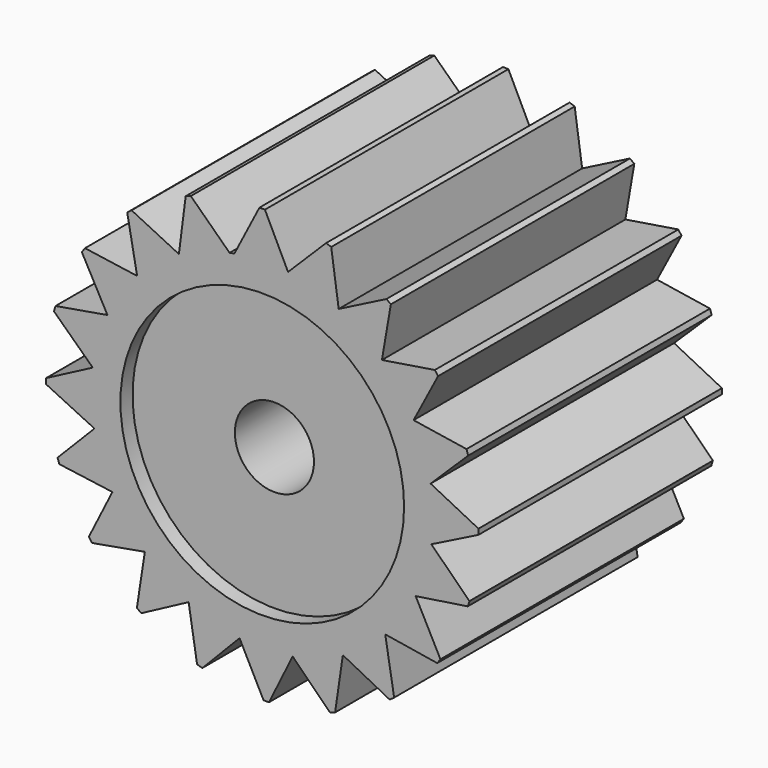
from build123d import *

# Parameters (mm, degrees)
F1_DEPTH = 25.4
F2_SIZE  = 0.508
F3_R     = 3.302
F4_DEPTH = 25.401
F5_R     = 11.8393994815
F6_DEPTH = 1.27


# Not quite as in the source:
# - a pattern or mirror of a feature is missing from the dataset's text; its kind, count and spacing are read off the source's solid


with BuildPart() as f1:
    # F0 (on Front) → F1 (new body)
    with BuildSketch(Plane.XZ):
        with BuildLine():
            ThreePointArc((2.1955722256, 14.0049672679), (2.1389839725, 14.013721602), (2.0823608197, 14.0222472874))
            ThreePointArc((2.0823608197, 14.0222472874), (-0.1238177863, 14.1754828746), (-2.3269830694, 13.9837332414))
            ThreePointArc((-2.3269830694, 13.9837332414), (-2.5271600448, 13.9489464721), (-2.7268178935, 13.9112943233))
            ThreePointArc((-2.7268178935, 13.9112943233), (-4.8572204087, 13.3179223407), (-6.8694139522, 12.4004353764))
            ThreePointArc((-6.8694139522, 12.4004353764), (-6.9194470584, 12.3725865517), (-6.9693672664, 12.3445358551))
            ThreePointArc((-6.9693672664, 12.3445358551), (-8.7595213047, 11.1458706293), (-10.3473616978, 9.6897756149))
            ThreePointArc((-10.3473616978, 9.6897756149), (-10.3864172478, 9.6479004103), (-10.4253033325, 9.60586779))
            ThreePointArc((-10.4253033325, 9.60586779), (-11.7605415234, 7.9151316255), (-12.8241532244, 6.0415842004))
            ThreePointArc((-12.8241532244, 6.0415842004), (-12.8484524089, 5.9897342401), (-12.8725419575, 5.937786551))
            ThreePointArc((-12.8725419575, 5.937786551), (-13.6236736863, 3.9185661741), (-14.060147229, 1.8088409193))
            ThreePointArc((-14.060147229, 1.8088409193), (-14.067338987, 1.7520329324), (-14.0743012216, 1.6951963594))
            ThreePointArc((-14.0743012216, 1.6951963594), (-14.1686509384, -0.4571391014), (-13.9357554417, -2.5989162821))
            ThreePointArc((-13.9357554417, -2.5989162821), (-13.9251439365, -2.6551858539), (-13.914305228, -2.7114121035))
            ThreePointArc((-13.914305228, -2.7114121035), (-13.3427441511, -4.7886140051), (-12.4630133566, -6.7552160324))
            ThreePointArc((-12.4630133566, -6.7552160324), (-12.4356253016, -6.8055028418), (-12.4080343463, -6.8556786122))
            ThreePointArc((-12.4080343463, -6.8556786122), (-11.2258637152, -8.6567678391), (-9.7844157411, -10.2579166587))
            ThreePointArc((-9.7844157411, -10.2579166587), (-9.7429010602, -10.2973552188), (-9.7012274137, -10.3366257667))
            ThreePointArc((-9.7012274137, -10.3366257667), (-8.0228278321, -11.6873384117), (-6.1591295924, -12.768115297))
            ThreePointArc((-6.1591295924, -12.768115297), (-6.1075050275, -12.7928897404), (-6.0557808122, -12.8174554544))
            ThreePointArc((-6.0557808122, -12.8174554544), (-4.0435453838, -13.587103676), (-1.9379185041, -14.0429383479))
            ThreePointArc((-1.9379185041, -14.0429383479), (-1.8811789762, -14.0506516302), (-1.8244087549, -14.0581356612))
            ThreePointArc((-1.8244087549, -14.0581356612), (0.3269692188, -14.1722523511), (2.4707953718, -13.9590406477))
            ThreePointArc((2.4707953718, -13.9590406477), (2.5271600448, -13.9489464721), (2.5834834846, -13.9386247047))
            ThreePointArc((2.5834834846, -13.9386247047), (4.6658480019, -13.3861685331), (6.640448101, -12.5245396958))
            ThreePointArc((6.640448101, -12.5245396958), (6.6909843703, -12.4976147216), (6.7414114691, -12.4704858356))
            ThreePointArc((6.7414114691, -12.4704858356), (8.5532839071, -11.3049095519), (10.1676060468, -9.8782302489))
            ThreePointArc((10.1676060468, -9.8782302489), (10.2074242891, -9.8370795948), (10.2470759865, -9.7957684384))
            ThreePointArc((10.2470759865, -9.7957684384), (11.613149111, -8.1298470648), (12.7109999837, -6.2761552711))
            ThreePointArc((12.7109999837, -6.2761552711), (12.7362475956, -6.2247604577), (12.7612874022, -6.1732640808))
            ThreePointArc((12.7612874022, -6.1732640808), (13.5493871727, -4.1681833951), (14.0245445102, -2.0668325655))
            ThreePointArc((14.0245445102, -2.0668325655), (14.0327786658, -2.0101662842), (14.0407838617, -1.953467205))
            ThreePointArc((14.0407838617, -1.953467205), (14.1421732628, -0.9790714877), (14.1760236164, 0))
            ThreePointArc((14.1760236164, 0), (14.127220701, 1.1752790468), (13.9811479763, 2.3424659733))
            ThreePointArc((13.9811479763, 2.3424659733), (13.971571982, 2.3989209915), (13.9617680268, 2.4553368688))
            ThreePointArc((13.9617680268, 2.4553368688), (13.4284633772, 4.54268829), (12.5850092021, 6.5251198421))
            ThreePointArc((12.5850092021, 6.5251198421), (12.5585495807, 6.5759013071), (12.5318850533, 6.6265754793))
            ThreePointArc((12.5318850533, 6.6265754793), (11.3830014695, 8.4490782407), (9.971211222, 10.0764374825))
            ThreePointArc((9.971211222, 10.0764374825), (9.9304280671, 10.1166320471), (9.8894828868, 10.1566615482))
            ThreePointArc((9.8894828868, 10.1566615482), (8.2361802932, 11.5379798817), (6.3926513618, 12.652812104))
            ThreePointArc((6.3926513618, 12.652812104), (6.3414906367, 12.6785307539), (6.2902264434, 12.7040425402))
            ThreePointArc((6.2902264434, 12.7040425402), (4.2924696912, 13.5105273592), (2.1955722256, 14.0049672679))
        make_face()
        with BuildLine():
            Line((2.1528735086, 14.0923740697), (2.0823608197, 14.0222472874))
            ThreePointArc((2.0823608197, 14.0222472874), (2.1389839725, 14.013721602), (2.1955722256, 14.0049672679))
            Line((2.1955722256, 14.0049672679), (2.1528735086, 14.0923740697))
        make_face()
        with BuildLine():
            ThreePointArc((-2.3269830694, 13.9837332414), (-0.1238177863, 14.1754828746), (2.0823608197, 14.0222472874))
            Line((2.0823608197, 14.0222472874), (2.1528735086, 14.0923740697))
            Line((2.1528735086, 14.0923740697), (0, 18.4994336074))
            Line((0, 18.4994336074), (-2.3269830694, 13.9837332414))
        make_face()
        with BuildLine():
            Line((2.1528735086, 14.0923740697), (2.1955722256, 14.0049672679))
            ThreePointArc((2.1955722256, 14.0049672679), (4.2924696912, 13.5105273592), (6.2902264434, 12.7040425402))
            Line((6.2902264434, 12.7040425402), (6.3788757147, 12.7491103956))
            Line((6.3788757147, 12.7491103956), (5.6843062312, 17.6044797271))
            Line((5.6843062312, 17.6044797271), (2.1528735086, 14.0923740697))
        make_face()
        with BuildLine():
            ThreePointArc((-6.8694139522, 12.4004353764), (-4.8572204087, 13.3179223407), (-2.7268178935, 13.9112943233))
            Line((-2.7268178935, 13.9112943233), (-6.3271789338, 17.3837812496))
            Line((-6.3271789338, 17.3837812496), (-6.9567956084, 12.4431855297))
            Line((-6.9567956084, 12.4431855297), (-6.8694139522, 12.4004353764))
        make_face()
        with BuildLine():
            Line((6.3788757147, 12.7491103956), (6.2902264434, 12.7040425402))
            ThreePointArc((6.2902264434, 12.7040425402), (6.3414906367, 12.6785307539), (6.3926513618, 12.652812104))
            Line((6.3926513618, 12.652812104), (6.3788757147, 12.7491103956))
        make_face()
        with BuildLine():
            ThreePointArc((-6.9693672664, 12.3445358551), (-6.9194470584, 12.3725865517), (-6.8694139522, 12.4004353764))
            Line((-6.8694139522, 12.4004353764), (-6.9567956084, 12.4431855297))
            Line((-6.9567956084, 12.4431855297), (-6.9693672664, 12.3445358551))
        make_face()
        with BuildLine():
            Line((6.3788757147, 12.7491103956), (6.3926513618, 12.652812104))
            ThreePointArc((6.3926513618, 12.652812104), (8.2361802932, 11.5379798817), (9.8894828868, 10.1566615482))
            Line((9.8894828868, 10.1566615482), (9.9876915038, 10.1723099485))
            Line((9.9876915038, 10.1723099485), (10.8186289304, 15.0062091102))
            Line((10.8186289304, 15.0062091102), (6.3788757147, 12.7491103956))
        make_face()
        with BuildLine():
            ThreePointArc((-10.3473616978, 9.6897756149), (-8.7595213047, 11.1458706293), (-6.9693672664, 12.3445358551))
            Line((-6.9693672664, 12.3445358551), (-6.9567956084, 12.4431855297))
            Line((-6.9567956084, 12.4431855297), (-11.3625872992, 14.5986524605))
            Line((-11.3625872992, 14.5986524605), (-10.443651865, 9.7036079365))
            Line((-10.443651865, 9.7036079365), (-10.3473616978, 9.6897756149))
        make_face()
        with BuildLine():
            Line((9.9876915038, 10.1723099485), (9.8894828868, 10.1566615482))
            ThreePointArc((9.8894828868, 10.1566615482), (9.9304280671, 10.1166320471), (9.971211222, 10.0764374825))
            Line((9.971211222, 10.0764374825), (9.9876915038, 10.1723099485))
        make_face()
        with BuildLine():
            ThreePointArc((-10.4253033325, 9.60586779), (-10.3864172478, 9.6479004103), (-10.3473616978, 9.6897756149))
            Line((-10.3473616978, 9.6897756149), (-10.443651865, 9.7036079365))
            Line((-10.443651865, 9.7036079365), (-10.4253033325, 9.60586779))
        make_face()
        with BuildLine():
            Line((9.9876915038, 10.1723099485), (9.971211222, 10.0764374825))
            ThreePointArc((9.971211222, 10.0764374825), (11.3830014695, 8.4490782407), (12.5318850533, 6.6265754793))
            Line((12.5318850533, 6.6265754793), (12.6301508676, 6.6112903677))
            Line((12.6301508676, 6.6112903677), (14.9061980753, 10.9560167366))
            Line((14.9061980753, 10.9560167366), (9.9876915038, 10.1723099485))
        make_face()
        with BuildLine():
            ThreePointArc((-12.8241532244, 6.0415842004), (-11.7605415234, 7.9151316255), (-10.4253033325, 9.60586779))
            Line((-10.4253033325, 9.60586779), (-10.443651865, 9.7036079365))
            Line((-10.443651865, 9.7036079365), (-15.2986115636, 10.4010349495))
            Line((-15.2986115636, 10.4010349495), (-12.9200353733, 6.0251603477))
            Line((-12.9200353733, 6.0251603477), (-12.8241532244, 6.0415842004))
        make_face()
        with BuildLine():
            Line((12.6301508676, 6.6112903677), (12.5318850533, 6.6265754793))
            ThreePointArc((12.5318850533, 6.6265754793), (12.5585495807, 6.5759013071), (12.5850092021, 6.5251198421))
            Line((12.5850092021, 6.5251198421), (12.6301508676, 6.6112903677))
        make_face()
        with BuildLine():
            ThreePointArc((-12.8725419575, 5.937786551), (-12.8484524089, 5.9897342401), (-12.8241532244, 6.0415842004))
            Line((-12.8241532244, 6.0415842004), (-12.9200353733, 6.0251603477))
            Line((-12.9200353733, 6.0251603477), (-12.8725419575, 5.937786551))
        make_face()
        with BuildLine():
            Line((12.6301508676, 6.6112903677), (12.5850092021, 6.5251198421))
            ThreePointArc((12.5850092021, 6.5251198421), (13.4284633772, 4.54268829), (13.9617680268, 2.4553368688))
            Line((13.9617680268, 2.4553368688), (14.0505833556, 2.4105971522))
            Line((14.0505833556, 2.4105971522), (17.5515220045, 5.8457778882))
            Line((17.5515220045, 5.8457778882), (12.6301508676, 6.6112903677))
        make_face()
        with BuildLine():
            ThreePointArc((-14.060147229, 1.8088409193), (-13.6236736863, 3.9185661741), (-12.8725419575, 5.937786551))
            Line((-12.8725419575, 5.937786551), (-12.9200353733, 6.0251603477))
            Line((-12.9200353733, 6.0251603477), (-17.7544227499, 5.1970680784))
            Line((-17.7544227499, 5.1970680784), (-14.146344308, 1.7637499777))
            Line((-14.146344308, 1.7637499777), (-14.060147229, 1.8088409193))
        make_face()
        with BuildLine():
            Line((14.0505833556, 2.4105971522), (13.9617680268, 2.4553368688))
            ThreePointArc((13.9617680268, 2.4553368688), (13.971571982, 2.3989209915), (13.9811479763, 2.3424659733))
            Line((13.9811479763, 2.3424659733), (14.0505833556, 2.4105971522))
        make_face()
        with BuildLine():
            ThreePointArc((-14.0743012216, 1.6951963594), (-14.067338987, 1.7520329324), (-14.060147229, 1.8088409193))
            Line((-14.060147229, 1.8088409193), (-14.146344308, 1.7637499777))
            Line((-14.146344308, 1.7637499777), (-14.0743012216, 1.6951963594))
        make_face()
        with BuildLine():
            Line((14.0505833556, 2.4105971522), (13.9811479763, 2.3424659733))
            ThreePointArc((13.9811479763, 2.3424659733), (14.127220701, 1.1752790468), (14.1760236164, 0))
            ThreePointArc((14.1760236164, 0), (14.1421732628, -0.9790714877), (14.0407838617, -1.953467205))
            Line((14.0407838617, -1.953467205), (14.1115554018, -2.0233327473))
            Line((14.1115554018, -2.0233327473), (18.4986531073, 0.1699323607))
            Line((18.4986531073, 0.1699323607), (14.0505833556, 2.4105971522))
        make_face()
        with BuildLine():
            ThreePointArc((-13.9357554417, -2.5989162821), (-14.1686509384, -0.4571391014), (-14.0743012216, 1.6951963594))
            Line((-14.0743012216, 1.6951963594), (-14.146344308, 1.7637499777))
            Line((-14.146344308, 1.7637499777), (-18.4924095024, -0.5097397272))
            Line((-18.4924095024, -0.5097397272), (-14.0039274753, -2.6683115505))
            Line((-14.0039274753, -2.6683115505), (-13.9357554417, -2.5989162821))
        make_face()
        with BuildLine():
            ThreePointArc((-13.914305228, -2.7114121035), (-13.9251439365, -2.6551858539), (-13.9357554417, -2.5989162821))
            Line((-13.9357554417, -2.5989162821), (-14.0039274753, -2.6683115505))
            Line((-14.0039274753, -2.6683115505), (-13.914305228, -2.7114121035))
        make_face()
        with BuildLine():
            Line((14.1115554018, -2.0233327473), (14.0407838617, -1.953467205))
            ThreePointArc((14.0407838617, -1.953467205), (14.0327786658, -2.0101662842), (14.0245445102, -2.0668325655))
            Line((14.0245445102, -2.0668325655), (14.1115554018, -2.0233327473))
        make_face()
        with BuildLine():
            Line((17.6559519668, -5.5223549269), (14.1115554018, -2.0233327473))
            Line((14.1115554018, -2.0233327473), (14.0245445102, -2.0668325655))
            ThreePointArc((14.0245445102, -2.0668325655), (13.5493871727, -4.1681833951), (12.7612874022, -6.1732640808))
            Line((12.7612874022, -6.1732640808), (12.8071676719, -6.261495627))
            Line((12.8071676719, -6.261495627), (17.6559519668, -5.5223549269))
        make_face()
        with BuildLine():
            ThreePointArc((-12.4630133566, -6.7552160324), (-13.3427441511, -4.7886140051), (-13.914305228, -2.7114121035))
            Line((-13.914305228, -2.7114121035), (-14.0039274753, -2.6683115505))
            Line((-14.0039274753, -2.6683115505), (-17.4411681098, -6.1672278017))
            Line((-17.4411681098, -6.1672278017), (-12.5065643779, -6.8422013069))
            Line((-12.5065643779, -6.8422013069), (-12.4630133566, -6.7552160324))
        make_face()
        with BuildLine():
            ThreePointArc((-12.4080343463, -6.8556786122), (-12.4356253016, -6.8055028418), (-12.4630133566, -6.7552160324))
            Line((-12.4630133566, -6.7552160324), (-12.5065643779, -6.8422013069))
            Line((-12.5065643779, -6.8422013069), (-12.4080343463, -6.8556786122))
        make_face()
        with BuildLine():
            Line((12.8071676719, -6.261495627), (12.7612874022, -6.1732640808))
            ThreePointArc((12.7612874022, -6.1732640808), (12.7362475956, -6.2247604577), (12.7109999837, -6.2761552711))
            Line((12.7109999837, -6.2761552711), (12.8071676719, -6.261495627))
        make_face()
        with BuildLine():
            Line((15.1049539068, -10.6803282378), (12.8071676719, -6.261495627))
            Line((12.8071676719, -6.261495627), (12.7109999837, -6.2761552711))
            ThreePointArc((12.7109999837, -6.2761552711), (11.613149111, -8.1298470648), (10.2470759865, -9.7957684384))
            Line((10.2470759865, -9.7957684384), (10.2636258527, -9.8938291687))
            Line((10.2636258527, -9.8938291687), (15.1049539068, -10.6803282378))
        make_face()
        with BuildLine():
            ThreePointArc((-9.7844157411, -10.2579166587), (-11.2258637152, -8.6567678391), (-12.4080343463, -6.8556786122))
            Line((-12.4080343463, -6.8556786122), (-12.5065643779, -6.8422013069))
            Line((-12.5065643779, -6.8422013069), (-14.7024111525, -11.2280073964))
            Line((-14.7024111525, -11.2280073964), (-9.7991319827, -10.3540757023))
            Line((-9.7991319827, -10.3540757023), (-9.7844157411, -10.2579166587))
        make_face()
        with BuildLine():
            ThreePointArc((-9.7012274137, -10.3366257667), (-9.7429010602, -10.2973552188), (-9.7844157411, -10.2579166587))
            Line((-9.7844157411, -10.2579166587), (-9.7991319827, -10.3540757023))
            Line((-9.7991319827, -10.3540757023), (-9.7012274137, -10.3366257667))
        make_face()
        with BuildLine():
            Line((10.2636258527, -9.8938291687), (10.2470759865, -9.7957684384))
            ThreePointArc((10.2470759865, -9.7957684384), (10.2074242891, -9.8370795948), (10.1676060468, -9.8782302489))
            Line((10.1676060468, -9.8782302489), (10.2636258527, -9.8938291687))
        make_face()
        with BuildLine():
            Line((11.0924800636, -14.804929241), (10.2636258527, -9.8938291687))
            Line((10.2636258527, -9.8938291687), (10.1676060468, -9.8782302489))
            ThreePointArc((10.1676060468, -9.8782302489), (8.5532839071, -11.3049095519), (6.7414114691, -12.4704858356))
            Line((6.7414114691, -12.4704858356), (6.7270296539, -12.5688879102))
            Line((6.7270296539, -12.5688879102), (11.0924800636, -14.804929241))
        make_face()
        with BuildLine():
            ThreePointArc((-6.1591295924, -12.768115297), (-8.0228278321, -11.6873384117), (-9.7012274137, -10.3366257667))
            Line((-9.7012274137, -10.3366257667), (-9.7991319827, -10.3540757023))
            Line((-9.7991319827, -10.3540757023), (-10.5411263289, -15.2024241328))
            Line((-10.5411263289, -15.2024241328), (-6.1435871882, -12.8641442671))
            Line((-6.1435871882, -12.8641442671), (-6.1591295924, -12.768115297))
        make_face()
        with BuildLine():
            ThreePointArc((-6.0557808122, -12.8174554544), (-6.1075050275, -12.7928897404), (-6.1591295924, -12.768115297))
            Line((-6.1591295924, -12.768115297), (-6.1435871882, -12.8641442671))
            Line((-6.1435871882, -12.8641442671), (-6.0557808122, -12.8174554544))
        make_face()
        with BuildLine():
            Line((6.7270296539, -12.5688879102), (6.7414114691, -12.4704858356))
            ThreePointArc((6.7414114691, -12.4704858356), (6.6909843703, -12.4976147216), (6.640448101, -12.5245396958))
            Line((6.640448101, -12.5245396958), (6.7270296539, -12.5688879102))
        make_face()
        with BuildLine():
            Line((6.0067562729, -17.4970832675), (6.7270296539, -12.5688879102))
            Line((6.7270296539, -12.5688879102), (6.640448101, -12.5245396958))
            ThreePointArc((6.640448101, -12.5245396958), (4.6658480019, -13.3861685331), (2.5834834846, -13.9386247047))
            Line((2.5834834846, -13.9386247047), (2.5395614967, -14.0278472571))
            Line((2.5395614967, -14.0278472571), (6.0067562729, -17.4970832675))
        make_face()
        with BuildLine():
            ThreePointArc((-1.9379185041, -14.0429383479), (-4.0435453838, -13.587103676), (-6.0557808122, -12.8174554544))
            Line((-6.0557808122, -12.8174554544), (-6.1435871882, -12.8641442671))
            Line((-6.1435871882, -12.8641442671), (-5.359937641, -17.7059343802))
            Line((-5.359937641, -17.7059343802), (-1.8936212553, -14.1295459872))
            Line((-1.8936212553, -14.1295459872), (-1.9379185041, -14.0429383479))
        make_face()
        with BuildLine():
            ThreePointArc((-1.8244087549, -14.0581356612), (-1.8811789762, -14.0506516302), (-1.9379185041, -14.0429383479))
            Line((-1.9379185041, -14.0429383479), (-1.8936212553, -14.1295459872))
            Line((-1.8936212553, -14.1295459872), (-1.8244087549, -14.0581356612))
        make_face()
        with BuildLine():
            Line((2.5395614967, -14.0278472571), (2.5834834846, -13.9386247047))
            ThreePointArc((2.5834834846, -13.9386247047), (2.5271600448, -13.9489464721), (2.4707953718, -13.9590406477))
            Line((2.4707953718, -13.9590406477), (2.5395614967, -14.0278472571))
        make_face()
        with BuildLine():
            Line((0.3398503824, -18.4963116732), (2.5395614967, -14.0278472571))
            Line((2.5395614967, -14.0278472571), (2.4707953718, -13.9590406477))
            ThreePointArc((2.4707953718, -13.9590406477), (0.3269692188, -14.1722523511), (-1.8244087549, -14.0581356612))
            Line((-1.8244087549, -14.0581356612), (-1.8936212553, -14.1295459872))
            Line((-1.8936212553, -14.1295459872), (0.3398503824, -18.4963116732))
        make_face()
    extrude(amount=F1_DEPTH)

    # F2
    f2_edges = [f1.edges().sort_by_distance(p)[0] for p in [
        (0, -12.7, 18.499434),
        (5.684306, -12.7, 17.60448),
        (10.818629, -12.7, 15.006209),
        (14.906198, -12.7, 10.956017),
        (17.551522, -12.7, 5.845778),
        (18.498653, -12.7, 0.169932),
        (17.655952, -12.7, -5.522355),
        (15.104954, -12.7, -10.680328),
        (11.09248, -12.7, -14.804929),
        (6.006756, -12.7, -17.497083),
        (0.33985, -12.7, -18.496312),
        (-5.359938, -12.7, -17.705934),
        (-10.541126, -12.7, -15.202424),
        (-14.702411, -12.7, -11.228007),
        (-17.441168, -12.7, -6.167228),
        (-18.49241, -12.7, -0.50974),
        (-17.754423, -12.7, 5.197068),
        (-15.298612, -12.7, 10.401035),
        (-11.362587, -12.7, 14.598652),
        (-6.327179, -12.7, 17.383781),
    ]]
    chamfer(f2_edges, length=F2_SIZE)

    # F3 (on face) → F4 (cut, through all)
    with BuildSketch(Plane.XZ.offset(25.4)):
        Circle(F3_R)
    extrude(amount=-F4_DEPTH, mode=Mode.SUBTRACT)

    # F5 (on face) → F6 (cut)
    with BuildSketch(Plane.XZ.offset(25.4)):
        Circle(F5_R)
    f6 = extrude(amount=-F6_DEPTH, mode=Mode.SUBTRACT)

    # F6_copies: F6 across plane
    add(f6.mirror(Plane.ZX.offset(-12.7)), mode=Mode.SUBTRACT)


solid = f1.part
